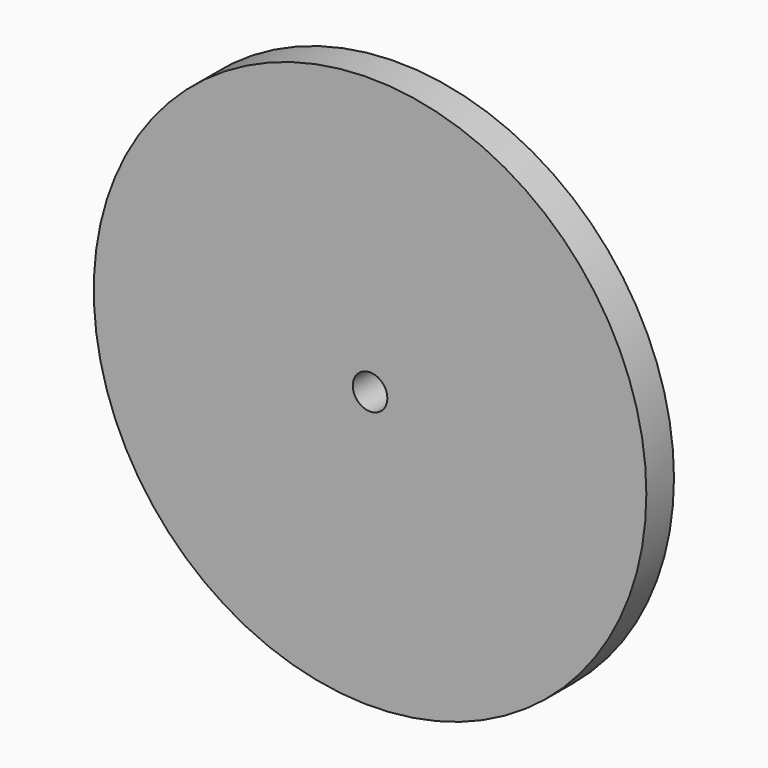
from build123d import *

# Parameters (mm, degrees)
F0_R     = 25.4
F0_R_2   = 22.86
F0_R_3   = 12.7
F0_R_4   = 1.5875
F1_DEPTH = 3.175


# Not quite as in the source:
# - a length typed as a fraction of an inch, garbled in the dataset ("3 / 203.2 mm" for 3/8 in), is restored
# - a feature names something its author has since deleted; it is built from what else it names


with BuildPart() as f1:
    # F0 (on Front) → F1 (new body)
    with BuildSketch(Plane.XZ):
        Circle(F0_R)
        Circle(F0_R_2, mode=Mode.SUBTRACT)
        Circle(F0_R_2)
        Circle(F0_R_3, mode=Mode.SUBTRACT)
        Circle(F0_R_3)
        Circle(F0_R_4, mode=Mode.SUBTRACT)
    extrude(amount=F1_DEPTH)


solid = f1.part
